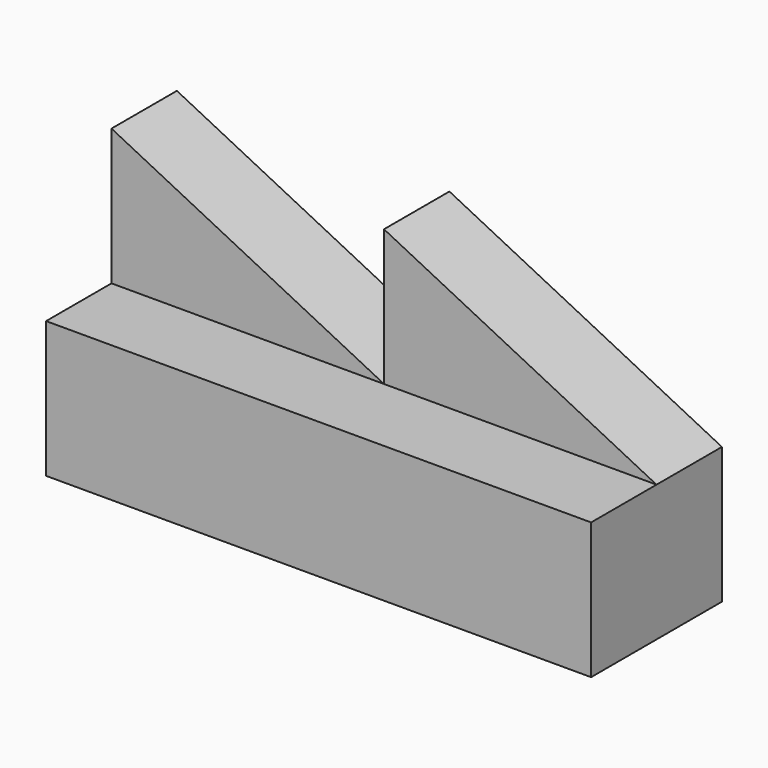
from build123d import *

# Parameters (mm, degrees)
F1_DEPTH = 38.1
F2_DEPTH = 19.05


# Not quite as in the source:
# - a length typed as a fraction of an inch, garbled in the dataset ("3 / 203.2 mm" for 3/8 in), is restored


with BuildPart() as f1:
    # F0 (on Front) → F1 (new body)
    with BuildSketch(Plane.XZ):
        Polygon((-63.5, 9.3406075202), (-63.5, -22.4093924798), (63.5, -22.4093924798), (63.5, 9.3406075202), (0, 9.3406075202), align=None)
    extrude(amount=F1_DEPTH)

    # F0 (on Front) → F2 (join)
    with BuildSketch(Plane.XZ):
        Polygon((-63.5, 41.0906075202), (-63.5, 9.3406075202), (0, 9.3406075202), align=None)
        Polygon((0, 9.3406075202), (63.5, 9.3406075202), (0, 41.0906075202), align=None)
    extrude(amount=F2_DEPTH)


solid = f1.part
